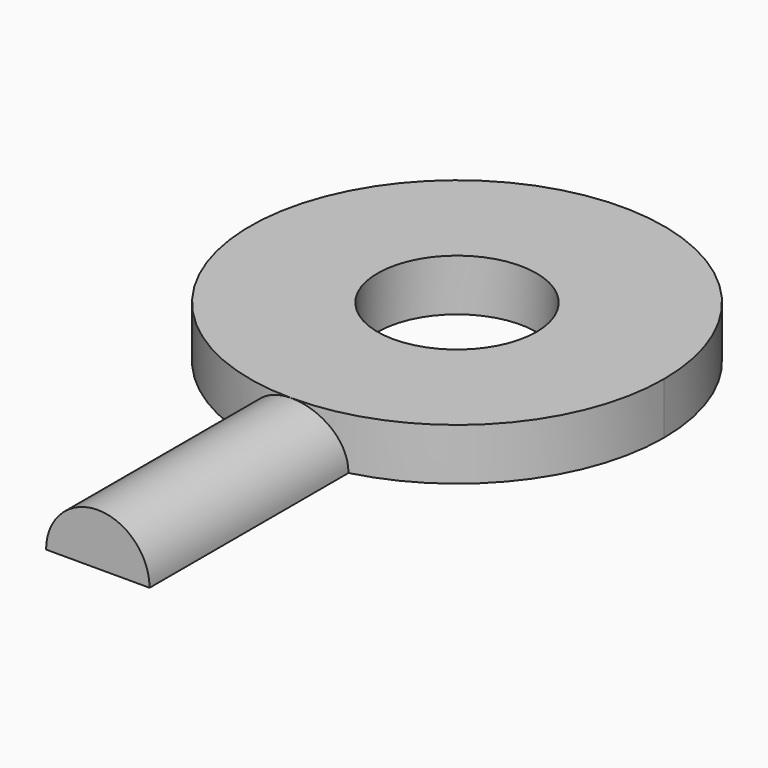
from build123d import *
from build123d import SkipClean  # not in build123d's __all__

# Parameters (mm, degrees)
F1_DEPTH = 50
F2_R     = 28
F2_R_2   = 10.75
F3_DEPTH = 7


with BuildPart() as f1:
    # F0 (on Front) → F1 (new body)
    with BuildSketch(Plane.XZ):
        with BuildLine():
            Line((-2, 0), (0, 0))
            Line((0, 0), (10, 0))
            Line((10, 0), (12, 0))
            ThreePointArc((12, 0), (5, 7), (-2, 0))
        make_face()
    extrude(amount=F1_DEPTH)

    # F2 (on Top) → F3 (join)
    with BuildSketch(Plane.XY):
        with Locations((5, 10.75)):
            Circle(F2_R)
        with Locations((5, 10.75)):
            Circle(F2_R_2, mode=Mode.SUBTRACT)
    with SkipClean():  # cleaning this boolean's faces spoils the solid; the shape is the same uncleaned
        extrude(amount=F3_DEPTH)


solid = f1.part
